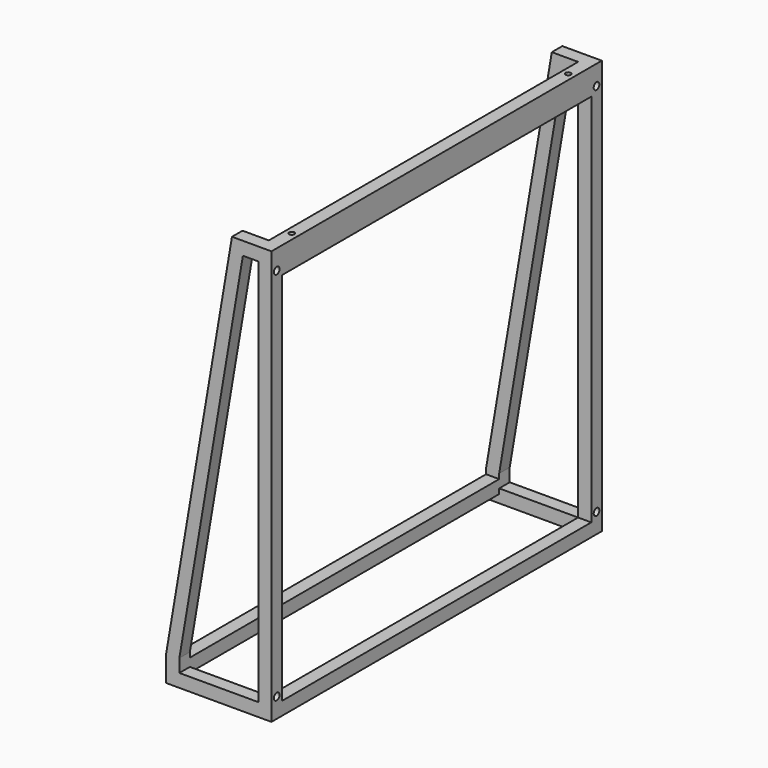
from build123d import *

# Parameters (mm, degrees)
F1_DEPTH = 12.7
F2_W     = 12.7
F2_H     = 12.7
F3_DEPTH = 373.29999
F5_DEPTH = 12.7
F7_D     = 6.8
F7_DEPTH = 15.75
F7_TIP   = 2.0429261047
F9_D     = 5.1054
F9_DEPTH = 30.48
F9_TIP   = 1.5338169022


# Not quite as in the source:
# - a feature names something its author has since deleted; it is built from what else it names


with BuildPart() as f1:
    # F0 (on Front) → F1 (new body)
    with BuildSketch(Plane.XZ):
        Polygon((0, 25.4), (0, 0), (101.6, 0), (101.6, 387.3), (101.6, 400), (63.5, 400), align=None)
        Polygon((88.9, 387.3), (88.9, 12.7), (12.7, 12.7), (12.7, 25.4), (74.047170315, 387.3), align=None, mode=Mode.SUBTRACT)
    extrude(amount=F1_DEPTH)

    # F2 (on face) → F3 (join)
    with BuildSketch(Plane(origin=(0, 0, 0), x_dir=(-1, 0, 0), z_dir=(0, 1, 0))):
        with Locations((-95.25, 6.35)):
            Rectangle(F2_W, F2_H)
        with Locations((-95.25, 393.65)):
            Rectangle(F2_W, F2_H)
        Polygon((-12.7, 20.574), (-12.7, 12.7), (-12.7, 7.874), (0, 7.874), (0, 20.574), align=None)
        with Locations((-95.25, 380.95)):
            Rectangle(F2_W, F2_H)
    extrude(amount=F3_DEPTH)

    # F4 (on face) → F5 (join)
    with BuildSketch(Plane(origin=(0, 373.29999, 0), x_dir=(-1, 0, 0), z_dir=(0, 1, 0))):
        Polygon((-101.6, 374.6), (-101.6, 12.7), (-88.9, 12.7), (-88.9, 239.3), (-88.9, 374.6), align=None)
        Polygon((-101.6, 12.7), (-101.6, 0), (0, 0), (0, 25.4), (-63.5, 400), (-88.9, 400), (-88.9, 387.3), (-74.047170315, 387.3), (-12.7, 25.4), (-12.7, 12.7), (-88.9, 12.7), align=None)
        Polygon((-101.6, 400), (-101.6, 374.6), (-88.9, 374.6), (-88.9, 387.3), (-88.9, 400), align=None)
    extrude(amount=F5_DEPTH)

    # F7
    with Locations(Plane.YZ.offset(101.6)):
        with Locations((-6.35, 19), (-6.35, 381), (379.64999, 381), (379.64999, 19)):
            Hole(F7_D / 2, depth=F7_DEPTH)
            with Locations((0, 0, -(F7_DEPTH + F7_TIP / 2))):  # 118° drill point
                Cone(0, F7_D / 2, F7_TIP, mode=Mode.SUBTRACT)

    # F9
    with Locations(Plane.XY.offset(400)):
        with Locations((95.25, 353.4243106842), (95.25, 19.8756793158)):
            Hole(F9_D / 2, depth=F9_DEPTH)
            with Locations((0, 0, -(F9_DEPTH + F9_TIP / 2))):  # 118° drill point
                Cone(0, F9_D / 2, F9_TIP, mode=Mode.SUBTRACT)


solid = f1.part
